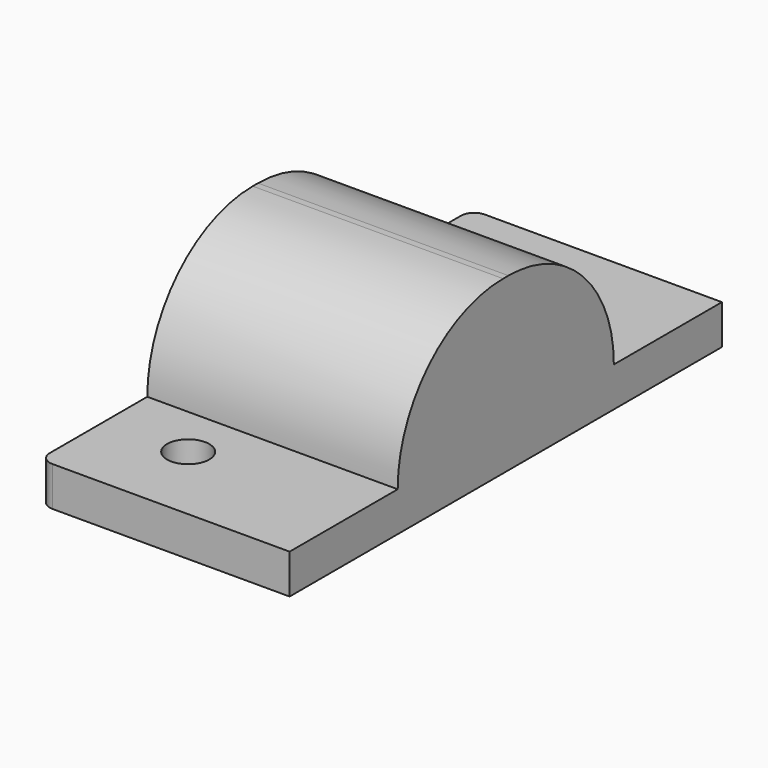
from build123d import *

# Parameters (mm, degrees)
F0_W     = 19
F0_H     = 41
F0_R     = 1.6
F1_DEPTH = 3
F2_R     = 1
F3_W     = 19
F3_H     = 20.5
F4_DEPTH = 10
F5_R     = 9.99999


# Not quite as in the source:
# - a fillet or chamfer is up to 0.001 mm smaller than in the source, because OpenCascade refuses the exact size


with BuildPart() as f1:
    # F0 (on Top) → F1 (new body)
    with BuildSketch(Plane.XY):
        with Locations((-9.5, 0)):
            Rectangle(F0_W, F0_H)
        with Locations((-12.7, -14.25)):
            Circle(F0_R, mode=Mode.SUBTRACT)
        with Locations((-12.7, 14.25)):
            Circle(F0_R, mode=Mode.SUBTRACT)
    extrude(amount=F1_DEPTH)

    # F2
    f2_edges = [f1.edges().sort_by_distance(p)[0] for p in [
        (-19, -20.5, 1.5),
        (-19, 20.5, 1.5),
    ]]
    fillet(f2_edges, radius=F2_R)

    # F3 (on face) → F4 (join)
    with BuildSketch(Plane.XY.offset(3)):
        with Locations((-9.5, 0)):
            Rectangle(F3_W, F3_H)
    extrude(amount=F4_DEPTH)

    # F5 (radius 10 in the source; OpenCascade refuses exactly that, so slightly less here)
    f5_edges = [f1.edges().sort_by_distance(p)[0] for p in [
        (-9.5, 10.25, 13),
        (-9.5, -10.25, 13),
    ]]
    fillet(f5_edges, radius=F5_R)


solid = f1.part
